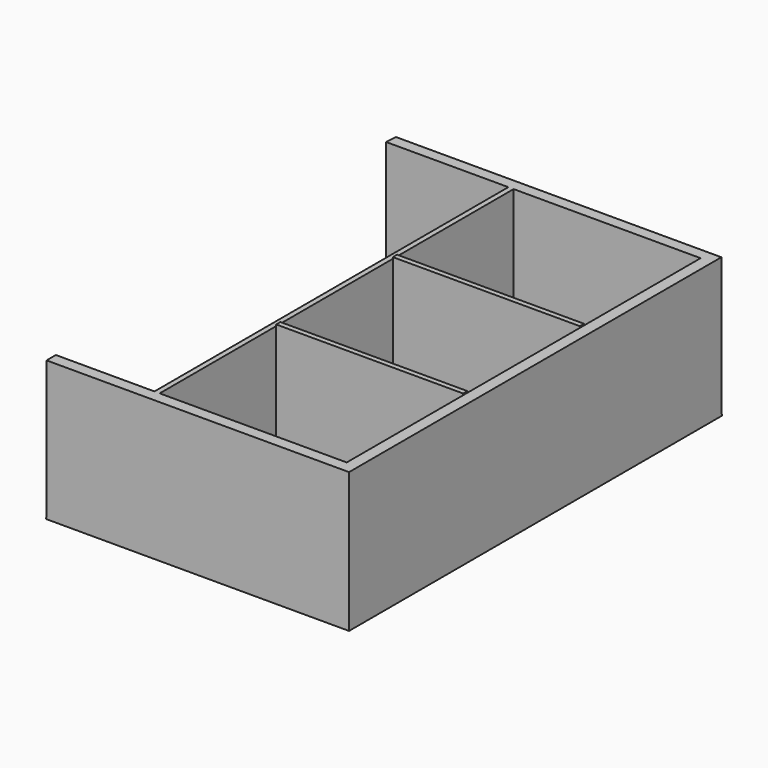
from build123d import *

# Parameters (mm, degrees)
F1_DEPTH  = 25
F3_DEPTH  = 25
F4_DEPTH  = 2400
F5_W      = 90
F5_H      = 7592.9608154297
F6_DEPTH  = 2400
F7_R      = 100
F8_DEPTH  = 500
F9_W      = 3210
F9_H      = 90
F10_DEPTH = 2400


with BuildPart() as f1:
    # F0 (on Top) → F1 (new body)
    with BuildSketch(Plane.XY):
        Polygon((2126.3071060181, 7160.2022171021), (-3073.6928939819, 7160.2022171021), (-3473.6928939819, 7160.2022171021), (-3473.6928939819, 4960.2022171021), (-3073.6928939819, 4960.2022171021), (-3073.6928939819, -839.7977828979), (2126.3071060181, -839.7977828979), align=None)
    extrude(amount=F1_DEPTH)

    # F7 (on face) → F8 (cut)
    with BuildSketch(Plane.XY):
        with Locations((-73.6928939819, 2160.2022171021)):
            Circle(F7_R)
    extrude(amount=F8_DEPTH, mode=Mode.SUBTRACT)


with BuildPart() as f3:
    # F2 (on face) → F3 (new body)
    with BuildSketch(Plane.XY):
        Polygon((2126.3071060181, 7148.1630325317), (-3457.8437805176, 7148.1630325317), (-3473.6928939819, 6953.1630325317), (1926.3071060181, 6953.1630325317), (1926.3071060181, -639.7977828979), (-3065.9193992615, -639.7977828979), (-3065.9193992615, -839.7977828979), (2126.3071060181, -839.7977828979), align=None)
    extrude(amount=F3_DEPTH)


with BuildPart() as f4:
    # F2 (on face) → F4 (new body)
    with BuildSketch(Plane.XY):
        Polygon((2126.3071060181, 7148.1630325317), (-3457.8437805176, 7148.1630325317), (-3473.6928939819, 6953.1630325317), (1926.3071060181, 6953.1630325317), (1926.3071060181, -639.7977828979), (-3065.9193992615, -639.7977828979), (-3065.9193992615, -839.7977828979), (2126.3071060181, -839.7977828979), align=None)
    extrude(amount=F4_DEPTH)

    # F5 (on face) → F6 (join)
    with BuildSketch(Plane.XY):
        with Locations((-1328.6928939819, 3156.6826248169)):
            Rectangle(F5_W, F5_H)
    extrude(amount=F6_DEPTH)


with BuildPart() as f10:
    # F9 (on face) → F10 (new body)
    with BuildSketch(Plane.XY.offset(25)):
        with Locations((321.3071060181, 1905.2022171021)):
            Rectangle(F9_W, F9_H)
    extrude(amount=F10_DEPTH)


with BuildPart() as f10b:
    # F9 (on face) → F10, piece 2 (new body)
    with BuildSketch(Plane.XY.offset(25)):
        with Locations((321.3071060181, 4408.1630325317)):
            Rectangle(F9_W, F9_H)
    extrude(amount=F10_DEPTH)


solid = Compound([f1.part, f3.part, f4.part, f10.part, f10b.part])
